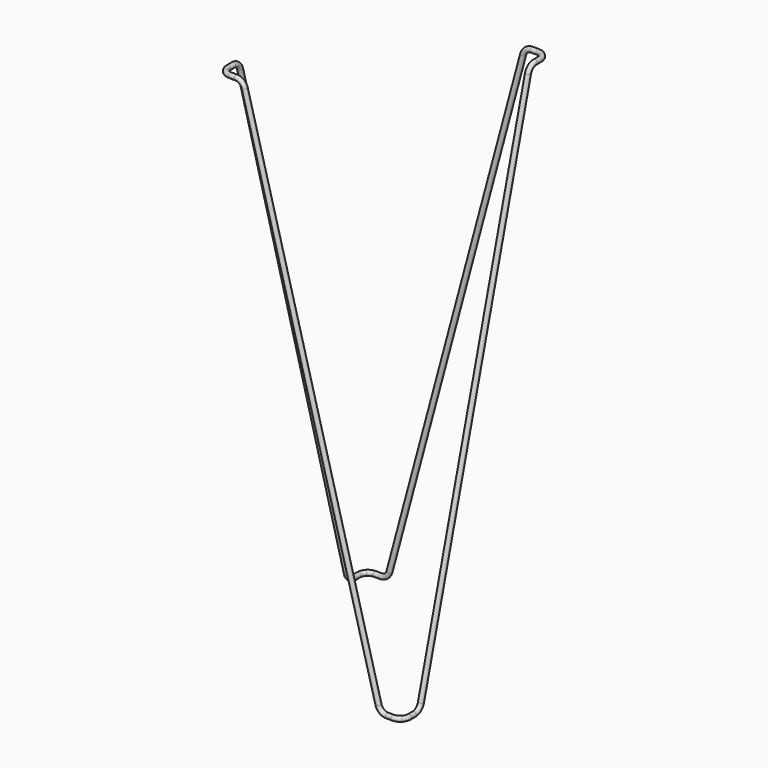
from build123d import *

# Parameters (mm, degrees)
F7_R            = 4
F8_COPIES_COUNT = 2


# Not quite as in the source:
# - a feature of the source that left no trace in its solid (it failed there, or was rolled back) is left out
# - a pattern or mirror of a feature is missing from the dataset's text; its kind, count and spacing are read off the source's solid


with BuildPart() as f8:
    # F8: sweep along a path in F6, F3, F5, F2, F6
    with BuildLine(Plane.XY) as f8_path:
        ThreePointArc((295.6066017178, 4.3933982822), (290.7402514855, 1.1418070123), (285, 0))
        Line((285, 0), (275.3883116029, 0))
    with BuildLine(Plane.XZ) as f8_path_2:
        ThreePointArc((275.3883116029, 0), (266.2568901678, 3.0996998956), (260.8994242086, 11.1177143235))
        Line((260.8994242086, 11.1177143235), (39.1005757914, 838.8822856765))
        ThreePointArc((39.1005757914, 838.8822856765), (33.7431098322, 846.9003001044), (24.6116883971, 850))
    with BuildLine(Plane.XY.offset(850)) as f8_path_3:
        Line((24.6116883971, 0), (15, 0))
        ThreePointArc((15, 0), (4.3933982822, 4.3933982822), (0, 15))
        Line((0, 15), (0, 24.6116883971))
    with BuildLine(Plane.YZ) as f8_path_4:
        ThreePointArc((24.6116883971, 850), (33.7431098322, 846.9003001044), (39.1005757914, 838.8822856765))
        Line((39.1005757914, 838.8822856765), (260.8994242086, 11.1177143235))
        ThreePointArc((260.8994242086, 11.1177143235), (266.2568901678, 3.0996998956), (275.3883116029, 0))
    with BuildLine(Plane.XY) as f8_path_5:
        Line((0, 275.3883116029), (0, 285))
        ThreePointArc((0, 285), (1.1418070123, 290.7402514855), (4.3933982822, 295.6066017178))
    # F7 (on face) → F8 (sweep)
    with BuildSketch(Plane(origin=(150, 150, 0), x_dir=(0.7071067812, -0.7071067812, 0), z_dir=(-0.7071067812, -0.7071067812, 0))):
        with Locations((205.9188309204, 0)):
            Circle(F7_R)
    sweep(path=f8_path.line + f8_path_2.line + f8_path_3.line + f8_path_4.line + f8_path_5.line)

    # F8_copies: F8 ×2 about axis
    f8_copies_axis = Axis((150, 150, 0), (0, 0, 1))


with BuildPart() as f8_1:
    add(f8.part)
    for i in range(1, F8_COPIES_COUNT):
        add(f8.part.rotate(f8_copies_axis, i * 360 / F8_COPIES_COUNT))


solid = f8_1.part
